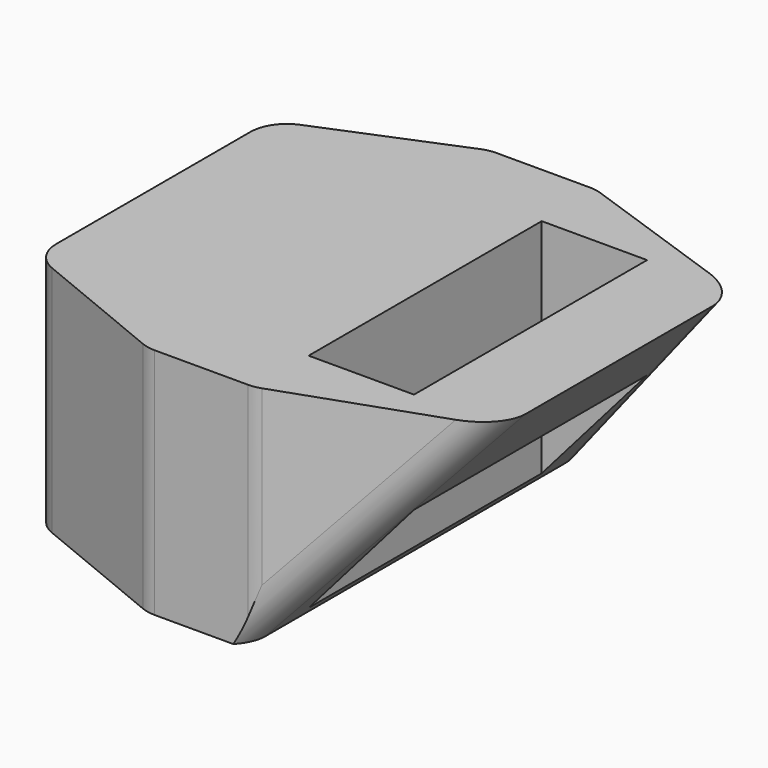
from build123d import *

# Parameters (mm, degrees)
F0_W        = 116.1797607577
F0_H        = 190.5
F1_DEPTH    = 304.8
F3_DEPTH    = 401.32
F4_DEPTH    = 942.34
F5_T1_DEPTH = 331.0069513468
F5_T3_DEPTH = 352.1111565483
F5_T5_DEPTH = 464.9612906349
F5_T7_DEPTH = 766.5905156751
F5_T9_DEPTH = 766.5905156751


# Not quite as in the source:
# - a fillet or chamfer that OpenCascade refuses, or shapes differently, is made with other operations: its cross-section is extruded or revolved along the edge and cut away or added


with BuildPart() as f1:
    # F0 (on Top) → F1 (new body)
    with BuildSketch(Plane.XY):
        Polygon((50.8, 190.5), (50.8, 279.4), (-88.9, 279.4), (-88.9, 190.5), (-88.9, 0), (0, 0), (50.8, 0), align=None)
        Polygon((188.6202392423, 231.1629162652), (50.8, 279.4), (50.8, 190.5), (188.6202392423, 190.5), align=None)
        Polygon((-88.9, 190.5), (-88.9, 279.4), (-304.8, 190.5), (-304.8, 0), (-188.6202392423, 0), (-88.9, 0), align=None)
        Polygon((304.8, 190.5), (188.6202392423, 231.1629162652), (188.6202392423, 190.5), align=None)
        with Locations((246.7101196212, 95.25)):
            Rectangle(F0_W, F0_H)
        Polygon((50.8, -190.5), (50.8, 0), (0, 0), (-88.9, 0), (-88.9, -190.5), (-88.9, -279.4), (50.8, -279.4), align=None)
        Polygon((-88.9, -190.5), (-88.9, 0), (-188.6202392423, 0), (-304.8, 0), (-304.8, -190.5), (-88.9, -279.4), align=None)
        with Locations((246.7101196212, -95.25)):
            Rectangle(F0_W, F0_H)
        Polygon((188.6202392423, -190.5), (50.8, -190.5), (50.8, -279.4), (188.6202392423, -231.1629162652), align=None)
        Polygon((304.8, -190.5), (188.6202392423, -190.5), (188.6202392423, -231.1629162652), align=None)
    extrude(amount=F1_DEPTH)

    # F2 (on Front) → F3 (cut)
    with BuildSketch(Plane.XZ):
        Polygon((306.468307972, 307.1446120739), (38.1901785731, 0), (-147.3951488733, -79.8071026802), (42.6088683307, 0), (5.996810738, -19.8390558362), (306.468307972, -19.8390558362), align=None)
    extrude(amount=-F3_DEPTH, mode=Mode.SUBTRACT)

    # F2 (on Front) → F4 (cut)
    with BuildSketch(Plane.XZ):
        Polygon((306.468307972, 307.1446120739), (38.1901785731, 0), (-147.3951488733, -79.8071026802), (42.6088683307, 0), (5.996810738, -19.8390558362), (306.468307972, -19.8390558362), align=None)
    extrude(amount=F4_DEPTH, mode=Mode.SUBTRACT)

    # F5: fillet of radius 47.8312768991 on 8 edges, made by hand

    # F5_s2 → F5_t1 (cut)
    with BuildSketch(Plane.XY.offset(-5.8851483368)):
        with BuildLine():
            ThreePointArc((42.671278796, 279.4), (50.6850979696, 278.7238898597), (58.4723614349, 276.7146734978))
            Line((58.4723614349, 276.7146734978), (50.8, 279.4))
            Line((50.8, 279.4), (42.671278796, 279.4))
        make_face()
        with BuildLine():
            ThreePointArc((58.4723614349, -276.7146734978), (50.6850979696, -278.7238898597), (42.671278796, -279.4))
            Line((42.671278796, -279.4), (50.8, -279.4))
            Line((50.8, -279.4), (58.4723614349, -276.7146734978))
        make_face()
    extrude(amount=F5_T1_DEPTH, mode=Mode.SUBTRACT)

    # F5_s4 → F5_t3 (cut)
    with BuildSketch(Plane.XY.offset(-23.6555782741)):
        with BuildLine():
            ThreePointArc((-97.6495180547, 275.7972572716), (-88.7201117415, 278.4906706018), (-79.4377686903, 279.4))
            Line((-79.4377686903, 279.4), (-88.9, 279.4))
            Line((-88.9, 279.4), (-97.6495180547, 275.7972572716))
        make_face()
        with BuildLine():
            ThreePointArc((-79.4377686903, -279.4), (-88.7201117415, -278.4906706018), (-97.6495180547, -275.7972572716))
            Line((-97.6495180547, -275.7972572716), (-88.9, -279.4))
            Line((-88.9, -279.4), (-79.4377686903, -279.4))
        make_face()
    extrude(amount=F5_T3_DEPTH, mode=Mode.SUBTRACT)

    # F5_s6 → F5_t5 (cut)
    with BuildSketch(Plane.XY.offset(-80.0806453175)):
        with BuildLine():
            ThreePointArc((-304.8, 158.467741873), (-296.7111580821, 185.0829614206), (-275.1804724653, 202.6962760437))
            Line((-275.1804724653, 202.6962760437), (-304.8, 190.5))
            Line((-304.8, 190.5), (-304.8, 158.467741873))
        make_face()
        with BuildLine():
            ThreePointArc((-275.1804724653, -202.6962760437), (-296.7111580821, -185.0829614206), (-304.8, -158.467741873))
            Line((-304.8, -158.467741873), (-304.8, -190.5))
            Line((-304.8, -190.5), (-275.1804724653, -202.6962760437))
        make_face()
    extrude(amount=F5_T5_DEPTH, mode=Mode.SUBTRACT)

    # F5_s8 → F5_t7 (cut)
    with BuildSketch(Plane(origin=(300.5564502803, -105.1947575981, 344.0992172359), x_dir=(-0.3303504247, -0.9438583564, 0), z_dir=(-0.6410735721, 0.2243757502, -0.7339483619))):
        with BuildLine():
            ThreePointArc((-280.4958263449, 79.454688834), (-270.4603992444, 50.1407879029), (-244.5651615788, 33.1275209877))
            Line((-244.5651615788, 33.1275209877), (-280.4958263449, 42.357459379))
            Line((-280.4958263449, 42.357459379), (-280.4958263449, 79.454688834))
        make_face()
    extrude(amount=F5_T7_DEPTH, mode=Mode.SUBTRACT)

    # F5_s10 → F5_t9 (cut)
    with BuildSketch(Plane(origin=(300.5564502803, 105.1947575981, 344.0992172359), x_dir=(0.3303504247, -0.9438583564, 0), z_dir=(-0.6410735721, -0.2243757502, -0.7339483619))):
        with BuildLine():
            ThreePointArc((280.4958263449, 79.454688834), (270.4603992444, 50.1407879029), (244.5651615788, 33.1275209877))
            Line((244.5651615788, 33.1275209877), (280.4958263449, 42.357459379))
            Line((280.4958263449, 42.357459379), (280.4958263449, 79.454688834))
        make_face()
    extrude(amount=F5_T9_DEPTH, mode=Mode.SUBTRACT)


solid = f1.part
